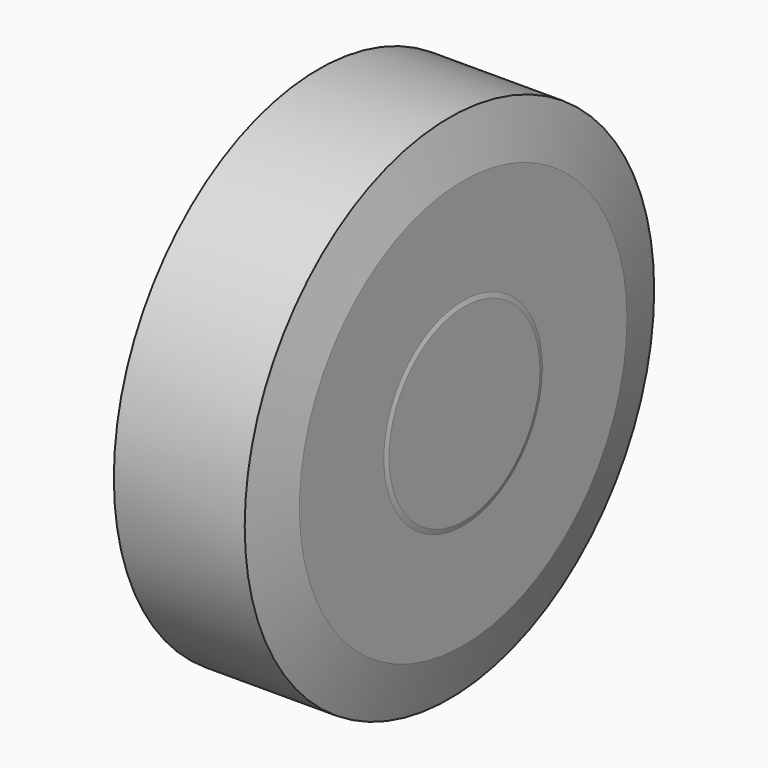
from build123d import *

# Parameters (mm, degrees)
F0_R     = 25.4
F1_DEPTH = 9.652
F2_R     = 4.7625
F3_DEPTH = 4.826
F4_DEPTH = 4.699
F6_DEPTH = 3.175
F7_R     = 6.35
F8_DEPTH = 1.524


# Not quite as in the source:
# - a fillet or chamfer that OpenCascade refuses, or shapes differently, is made with other operations: its cross-section is extruded or revolved along the edge and cut away or added


with BuildPart() as f1:
    # F0 (on Right) → F1 (new body)
    with BuildSketch(Plane.YZ):
        Circle(F0_R)
    extrude(amount=F1_DEPTH)

    # F2 (on face) → F3 (join)
    with BuildSketch(Plane.YZ.offset(9.652)):
        Circle(F2_R)
    extrude(amount=F3_DEPTH)

    # F4 (add): a face of the model
    f4_faces = [f1.faces().sort_by_distance(p)[0] for p in [
        (9.652, -24.6815795103, 0),
    ]]
    extrude(f4_faces, amount=F4_DEPTH)

    # F5: chamfer of 5.08 x 1.3611818976 on 2 edges, made by hand


with BuildPart() as f5_tool2:
    # F5_s3 → F5_t4 (revolve)
    with BuildSketch(Plane.XY):
        Polygon((14.351, 9.8425), (15.7121818976, 4.7625), (14.351, 4.7625), align=None)
    revolve(axis=Axis((14.351, 0, 0), (1, 0, 0)))

    split(bisect_by=Plane.YZ.offset(14.478), keep=Keep.BOTTOM)


with BuildPart() as f1_1:
    add(f1.part)

    # F5_t1: union F5_tool2
    add(f5_tool2.part)

    # F5_s6 → F5_t7 (revolve, cut)
    with BuildSketch(Plane.XY):
        Polygon((12.9898181024, 25.4), (14.351, 20.32), (14.351, 25.4), align=None)
    revolve(axis=Axis((14.351, 0, 0), (1, 0, 0)), mode=Mode.SUBTRACT)

    # F6 (cut): a face of the model
    f6_faces = [f1_1.faces().sort_by_distance(p)[0] for p in [
        (0, 0, 0),
    ]]
    extrude(f6_faces, amount=F6_DEPTH, mode=Mode.SUBTRACT)

    # F7 (on face) → F8 (join)
    with BuildSketch(Plane(origin=(0, 0, 0), x_dir=(0, -1, 0), z_dir=(-1, 0, 0))):
        Circle(F7_R)
    extrude(amount=F8_DEPTH)


solid = f1_1.part
